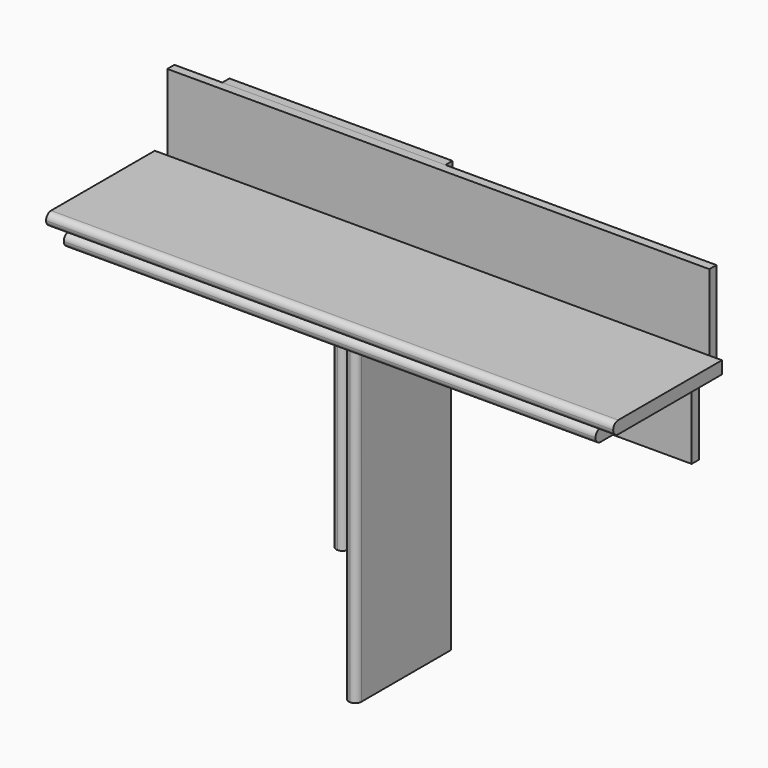
from build123d import *

# Parameters (mm, degrees)
F0_W      = 1219.2
F0_H      = 292.1
F1_DEPTH  = 26.924
F2_R      = 13.46199
F3_W      = 1165.352
F3_H      = 190.5
F4_DEPTH  = 19.05
F5_W      = 254
F5_H      = 711.2
F6_DEPTH  = 26.924
F7_W      = 254
F7_H      = 431.8
F8_DEPTH  = 26.924
F9_R      = 13.46199
F10_R     = 13.46199
F11_W     = 1143
F11_H     = 292.1
F12_DEPTH = 26.924
F13_R     = 13.46199
F14_W     = 1089.152
F14_H     = 190.5
F15_DEPTH = 19.05
F16_W     = 479.552
F16_H     = 190.5
F17_DEPTH = 19.05


# Not quite as in the source:
# - a fillet or chamfer is up to 0.001 mm smaller than in the source, because OpenCascade refuses the exact size


with BuildPart() as f1:
    # F0 (on Top) → F1 (new body)
    with BuildSketch(Plane.XY):
        with Locations((0, -146.05)):
            Rectangle(F0_W, F0_H)
    extrude(amount=F1_DEPTH)

    # F2 (radius 13.462 in the source; OpenCascade refuses exactly that, so slightly less here)
    f2_edges = [f1.edges().sort_by_distance(p)[0] for p in [
        (0, -292.1, 26.924),
        (0, -292.1, 0),
    ]]
    fillet(f2_edges, radius=F2_R)


with BuildPart() as f4:
    # F3 (on Front) → F4 (new body)
    with BuildSketch(Plane.XZ):
        with Locations((0, 95.25)):
            Rectangle(F3_W, F3_H)
    extrude(amount=-F4_DEPTH)


with BuildPart() as f6:
    # F5 (on Right) → F6 (new body)
    with BuildSketch(Plane.YZ):
        with Locations((-127, -355.6)):
            Rectangle(F5_W, F5_H)
    extrude(amount=F6_DEPTH)

    # F9 (radius 13.462 in the source; OpenCascade refuses exactly that, so slightly less here)
    f9_edges = [f6.edges().sort_by_distance(p)[0] for p in [
        (0, -254, -355.6),
        (26.924, -254, -355.6),
    ]]
    fillet(f9_edges, radius=F9_R)


with BuildPart() as f8:
    # F7 (on Right) → F8 (new body)
    with BuildSketch(Plane.YZ):
        with Locations((-127, -215.9)):
            Rectangle(F7_W, F7_H)
    extrude(amount=-F8_DEPTH)

    # F10 (radius 13.462 in the source; OpenCascade refuses exactly that, so slightly less here)
    f10_edges = [f8.edges().sort_by_distance(p)[0] for p in [
        (-26.924, -254, -215.9),
        (0, -254, -215.9),
        (-26.924, 0, -215.9),
        (0, 0, -215.9),
    ]]
    fillet(f10_edges, radius=F10_R)


with BuildPart() as f12:
    # F11 (on Top) → F12 (new body)
    with BuildSketch(Plane.XY):
        with Locations((0, -146.05)):
            Rectangle(F11_W, F11_H)
    extrude(amount=-F12_DEPTH)

    # F13 (radius 13.462 in the source; OpenCascade refuses exactly that, so slightly less here)
    f13_edges = [f12.edges().sort_by_distance(p)[0] for p in [
        (0, -292.1, 0),
        (0, -292.1, -26.924),
        (0, 0, -26.924),
        (0, 0, 0),
    ]]
    fillet(f13_edges, radius=F13_R)


with BuildPart() as f15:
    # F14 (on Front) → F15 (new body)
    with BuildSketch(Plane.XZ):
        with Locations((0, -95.25)):
            Rectangle(F14_W, F14_H)
    extrude(amount=-F15_DEPTH)


with BuildPart() as f17:
    # F16 (on face) → F17 (new body)
    with BuildSketch(Plane(origin=(0, 19.05, 0), x_dir=(-1, 0, 0), z_dir=(0, 1, 0))):
        with Locations((239.776, 95.25)):
            Rectangle(F16_W, F16_H)
    extrude(amount=F17_DEPTH)


solid = Compound([f1.part, f4.part, f6.part, f8.part, f12.part, f15.part, f17.part])
